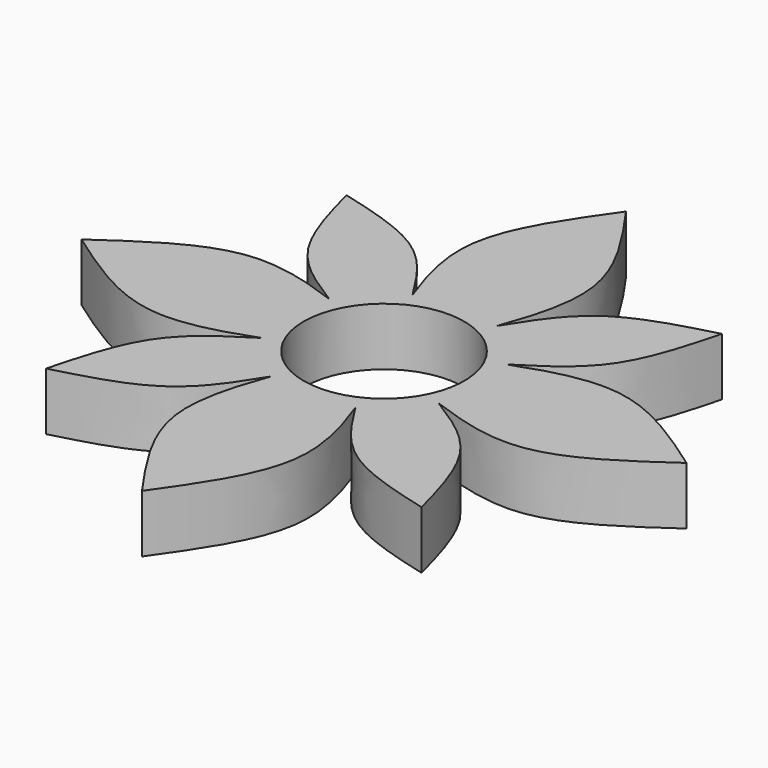
from build123d import *

# Parameters (mm, degrees)
F1_DEPTH = 8
F3_D     = 22.25


with BuildPart() as f1:
    # F0 (on Top) → F1 (new body)
    with BuildSketch(Plane.XY):
        with BuildLine():
            ThreePointArc((9.9471375726, 4.9819754226), (7.8665088435, 7.8666170375), (4.9818386126, 9.9472060921))
            ThreePointArc((4.9818386126, 9.9472060921), (0, 11.125), (-4.9818386126, 9.9472060921))
            ThreePointArc((-4.9818386126, 9.9472060921), (-7.8665088435, 7.8666170375), (-9.9471375726, 4.9819754226))
            ThreePointArc((-9.9471375726, 4.9819754226), (-11.125, 0), (-9.9471375726, -4.9819754226))
            ThreePointArc((-9.9471375726, -4.9819754226), (-7.8665088435, -7.8666170375), (-4.9818386126, -9.9472060921))
            ThreePointArc((-4.9818386126, -9.9472060921), (0, -11.125), (4.9818386126, -9.9472060921))
            ThreePointArc((4.9818386126, -9.9472060921), (7.8665088435, -7.8666170375), (9.9471375726, -4.9819754226))
            ThreePointArc((9.9471375726, -4.9819754226), (10.8265306192, -2.5596600853), (11.125, 0))
            ThreePointArc((11.125, 0), (10.8265306192, 2.5596600853), (9.9471375726, 4.9819754226))
        make_face()
        with BuildLine():
            add(Edge.make_bspline(
                [(4.9818386126, 9.9472060921), (5.2692870464, 10.7123686961), (5.5568645372, 11.4776931218), (5.8364125218, 12.242766493)],
                knots=[0, 0, 0, 0, 0.0701678859, 0.0701678859, 0.0701678859, 0.0701678859], degree=3))
            ThreePointArc((4.9818386126, 9.9472060921), (7.8665088435, 7.8666170375), (9.9471375726, 4.9819754226))
            add(Edge.make_bspline(
                [(9.9471375726, 4.9819754226), (10.7123016854, 5.2694244447), (11.4776275551, 5.5570012299), (12.2427023029, 5.8365471685)],
                knots=[1.11321e-05, 1.11321e-05, 1.11321e-05, 1.11321e-05, 0.0701791516, 0.0701791516, 0.0701791516, 0.0701791516], degree=3))
            ThreePointArc((12.2427023029, 5.8365471685), (9.5902820459, 9.5903875212), (5.8364125218, 12.242766493))
        make_face()
        with BuildLine():
            ThreePointArc((-4.9818386126, 9.9472060921), (0, 11.125), (4.9818386126, 9.9472060921))
            add(Edge.make_bspline(
                [(4.9818386126, 9.9472060921), (5.2692870464, 10.7123686961), (5.5568645372, 11.4776931218), (5.8364125218, 12.242766493)],
                knots=[0, 0, 0, 0, 0.0701678859, 0.0701678859, 0.0701678859, 0.0701678859], degree=3))
            ThreePointArc((5.8364125218, 12.242766493), (0, 13.5627815188), (-5.8364125218, 12.242766493))
            add(Edge.make_bspline(
                [(-4.9818386126, 9.9472060921), (-5.2692870464, 10.7123686961), (-5.5568645372, 11.4776931218), (-5.8364125218, 12.242766493)],
                knots=[0, 0, 0, 0, 0.0701678859, 0.0701678859, 0.0701678859, 0.0701678859], degree=3))
        make_face()
        with BuildLine():
            ThreePointArc((-9.9471375726, 4.9819754226), (-7.8665088435, 7.8666170375), (-4.9818386126, 9.9472060921))
            add(Edge.make_bspline(
                [(-4.9818386126, 9.9472060921), (-5.2692870464, 10.7123686961), (-5.5568645372, 11.4776931218), (-5.8364125218, 12.242766493)],
                knots=[0, 0, 0, 0, 0.0701678859, 0.0701678859, 0.0701678859, 0.0701678859], degree=3))
            ThreePointArc((-5.8364125218, 12.242766493), (-9.5902820459, 9.5903875212), (-12.2427023029, 5.8365471685))
            add(Edge.make_bspline(
                [(-9.9471375726, 4.9819754226), (-10.7123016854, 5.2694244447), (-11.4776275551, 5.5570012299), (-12.2427023029, 5.8365471685)],
                knots=[1.11321e-05, 1.11321e-05, 1.11321e-05, 1.11321e-05, 0.0701791516, 0.0701791516, 0.0701791516, 0.0701791516], degree=3))
        make_face()
        with BuildLine():
            add(Edge.make_bspline(
                [(9.9471375726, 4.9819754226), (10.7123016854, 5.2694244447), (11.4776275551, 5.5570012299), (12.2427023029, 5.8365471685)],
                knots=[1.11321e-05, 1.11321e-05, 1.11321e-05, 1.11321e-05, 0.0701791516, 0.0701791516, 0.0701791516, 0.0701791516], degree=3))
            ThreePointArc((9.9471375726, 4.9819754226), (10.8265306192, 2.5596600853), (11.125, 0))
            ThreePointArc((11.125, 0), (10.8265306192, -2.5596600853), (9.9471375726, -4.9819754226))
            add(Edge.make_bspline(
                [(9.9471375726, -4.9819754226), (10.7123016854, -5.2694244447), (11.4776275551, -5.5570012299), (12.2427023029, -5.8365471685)],
                knots=[1.11321e-05, 1.11321e-05, 1.11321e-05, 1.11321e-05, 0.0701791516, 0.0701791516, 0.0701791516, 0.0701791516], degree=3))
            ThreePointArc((12.2427023029, -5.8365471685), (12.2428068623, -5.8363278403), (12.2429114178, -5.8361085102))
            ThreePointArc((12.2429114178, -5.8361085102), (13.2286993926, -2.9917478013), (13.5627815188, 0))
            ThreePointArc((13.5627815188, 0), (13.2286993926, 2.9917478013), (12.2429114178, 5.8361085102))
            ThreePointArc((12.2429114178, 5.8361085102), (12.2428068623, 5.8363278403), (12.2427023029, 5.8365471685))
        make_face()
        with BuildLine():
            ThreePointArc((-5.8364125218, 12.242766493), (0, 13.5627815188), (5.8364125218, 12.242766493))
            add(Edge.make_bspline(
                [(5.8364125218, 12.242766493), (7.4881688325, 16.7633312564), (10.5639067692, 26.8820696151), (3.7644701713, 36.5283294837), (0, 41.8734326959)],
                knots=[0.0701678859, 0.0701678859, 0.0701678859, 0.0701678859, 0.484766648, 1, 1, 1, 1], degree=3))
            add(Edge.make_bspline(
                [(-5.8364125218, 12.242766493), (-7.4881688325, 16.7633312564), (-10.5639067692, 26.8820696151), (-3.7644701713, 36.5283294837), (0, 41.8734326959)],
                knots=[0.0701678859, 0.0701678859, 0.0701678859, 0.0701678859, 0.484766648, 1, 1, 1, 1], degree=3))
        make_face()
        Polygon((2.4637663324, 30.8732958237), (5.4101836661, 26.3272686725), (2.9464173337, 21.5025828357), (-2.4637663324, 21.2239241501), (-5.4101836661, 25.7699513014), (-2.9464173337, 30.5946371381), align=None, mode=Mode.SUBTRACT)
        with BuildLine():
            add(Edge.make_bspline(
                [(5.8364125218, 12.242766493), (7.8640126159, 15.4827332927), (12.1444054008, 22.3225093182), (21.2142960732, 24.7235177216), (25.987826083, 25.9871807669)],
                knots=[0, 0, 0, 0, 0.4736948677, 1, 1, 1, 1], degree=3))
            ThreePointArc((5.8364125218, 12.242766493), (9.5902820459, 9.5903875212), (12.2427023029, 5.8365471685))
            add(Edge.make_bspline(
                [(12.2427023029, 5.8365471685), (12.2434313303, 5.8368135433), (12.2441603575, 5.8370799108), (12.2448893845, 5.8373462711)],
                knots=[0.0701791516, 0.0701791516, 0.0701791516, 0.0701791516, 0.0702460136, 0.0702460136, 0.0702460136, 0.0702460136], degree=3))
            add(Edge.make_bspline(
                [(12.2448893845, 5.8373462711), (15.4842471687, 7.8644533679), (22.3230423426, 12.1447253647), (24.7240445028, 21.2136821375), (25.987826083, 25.9871807669)],
                knots=[9.63938e-05, 9.63938e-05, 9.63938e-05, 9.63938e-05, 0.4736948677, 1, 1, 1, 1], degree=3))
        make_face()
        with BuildLine():
            ThreePointArc((-9.9471375726, -4.9819754226), (-11.125, 0), (-9.9471375726, 4.9819754226))
            add(Edge.make_bspline(
                [(-9.9471375726, 4.9819754226), (-10.7123016854, 5.2694244447), (-11.4776275551, 5.5570012299), (-12.2427023029, 5.8365471685)],
                knots=[1.11321e-05, 1.11321e-05, 1.11321e-05, 1.11321e-05, 0.0701791516, 0.0701791516, 0.0701791516, 0.0701791516], degree=3))
            ThreePointArc((-12.2427023029, 5.8365471685), (-12.2428068623, 5.8363278403), (-12.2429114178, 5.8361085102))
            ThreePointArc((-12.2429114178, 5.8361085102), (-13.5627815188, 0), (-12.2429114178, -5.8361085102))
            ThreePointArc((-12.2429114178, -5.8361085102), (-12.2428068623, -5.8363278403), (-12.2427023029, -5.8365471685))
            add(Edge.make_bspline(
                [(-9.9471375726, -4.9819754226), (-10.7123016854, -5.2694244447), (-11.4776275551, -5.5570012299), (-12.2427023029, -5.8365471685)],
                knots=[1.11321e-05, 1.11321e-05, 1.11321e-05, 1.11321e-05, 0.0701791516, 0.0701791516, 0.0701791516, 0.0701791516], degree=3))
        make_face()
        with BuildLine():
            ThreePointArc((-12.2427023029, 5.8365471685), (-9.5902820459, 9.5903875212), (-5.8364125218, 12.242766493))
            add(Edge.make_bspline(
                [(-5.8364125218, 12.242766493), (-7.8640126159, 15.4827332927), (-12.1444054008, 22.3225093182), (-21.2142960732, 24.7235177216), (-25.987826083, 25.9871807669)],
                knots=[0, 0, 0, 0, 0.4736948677, 1, 1, 1, 1], degree=3))
            add(Edge.make_bspline(
                [(-12.2448893845, 5.8373462711), (-15.4842471687, 7.8644533679), (-22.3230423426, 12.1447253647), (-24.7240445028, 21.2136821375), (-25.987826083, 25.9871807669)],
                knots=[9.63938e-05, 9.63938e-05, 9.63938e-05, 9.63938e-05, 0.4736948677, 1, 1, 1, 1], degree=3))
            add(Edge.make_bspline(
                [(-12.2427023029, 5.8365471685), (-12.2434313303, 5.8368135433), (-12.2441603575, 5.8370799108), (-12.2448893845, 5.8373462711)],
                knots=[0.0701791516, 0.0701791516, 0.0701791516, 0.0701791516, 0.0702460136, 0.0702460136, 0.0702460136, 0.0702460136], degree=3))
        make_face()
        with BuildLine():
            add(Edge.make_bspline(
                [(12.2427023029, 5.8365471685), (12.2434313303, 5.8368135433), (12.2441603575, 5.8370799108), (12.2448893845, 5.8373462711)],
                knots=[0.0701791516, 0.0701791516, 0.0701791516, 0.0701791516, 0.0702460136, 0.0702460136, 0.0702460136, 0.0702460136], degree=3))
            ThreePointArc((12.2427023029, 5.8365471685), (12.2428068623, 5.8363278403), (12.2429114178, 5.8361085102))
            add(Edge.make_bspline(
                [(12.2429114178, 5.8361085102), (12.24357074, 5.8365210972), (12.2442300623, 5.8369336841), (12.2448893845, 5.8373462711)],
                knots=[0, 0, 0, 0, 9.63938e-05, 9.63938e-05, 9.63938e-05, 9.63938e-05], degree=3))
        make_face()
        with BuildLine():
            ThreePointArc((-4.9818386126, -9.9472060921), (-7.8665088435, -7.8666170375), (-9.9471375726, -4.9819754226))
            add(Edge.make_bspline(
                [(-9.9471375726, -4.9819754226), (-10.7123016854, -5.2694244447), (-11.4776275551, -5.5570012299), (-12.2427023029, -5.8365471685)],
                knots=[1.11321e-05, 1.11321e-05, 1.11321e-05, 1.11321e-05, 0.0701791516, 0.0701791516, 0.0701791516, 0.0701791516], degree=3))
            ThreePointArc((-12.2427023029, -5.8365471685), (-9.5902820459, -9.5903875212), (-5.8364125218, -12.242766493))
            add(Edge.make_bspline(
                [(-4.9818386126, -9.9472060921), (-5.2692870464, -10.7123686961), (-5.5568645372, -11.4776931218), (-5.8364125218, -12.242766493)],
                knots=[0, 0, 0, 0, 0.0701678859, 0.0701678859, 0.0701678859, 0.0701678859], degree=3))
        make_face()
        with BuildLine():
            ThreePointArc((-12.2429114178, 5.8361085102), (-12.2428068623, 5.8363278403), (-12.2427023029, 5.8365471685))
            add(Edge.make_bspline(
                [(-12.2427023029, 5.8365471685), (-12.2434313303, 5.8368135433), (-12.2441603575, 5.8370799108), (-12.2448893845, 5.8373462711)],
                knots=[0.0701791516, 0.0701791516, 0.0701791516, 0.0701791516, 0.0702460136, 0.0702460136, 0.0702460136, 0.0702460136], degree=3))
            add(Edge.make_bspline(
                [(-12.2429114178, 5.8361085102), (-12.24357074, 5.8365210972), (-12.2442300623, 5.8369336841), (-12.2448893845, 5.8373462711)],
                knots=[0, 0, 0, 0, 9.63938e-05, 9.63938e-05, 9.63938e-05, 9.63938e-05], degree=3))
        make_face()
        with BuildLine():
            add(Edge.make_bspline(
                [(9.9471375726, -4.9819754226), (10.7123016854, -5.2694244447), (11.4776275551, -5.5570012299), (12.2427023029, -5.8365471685)],
                knots=[1.11321e-05, 1.11321e-05, 1.11321e-05, 1.11321e-05, 0.0701791516, 0.0701791516, 0.0701791516, 0.0701791516], degree=3))
            ThreePointArc((9.9471375726, -4.9819754226), (7.8665088435, -7.8666170375), (4.9818386126, -9.9472060921))
            add(Edge.make_bspline(
                [(4.9818386126, -9.9472060921), (5.2692870464, -10.7123686961), (5.5568645372, -11.4776931218), (5.8364125218, -12.242766493)],
                knots=[0, 0, 0, 0, 0.0701678859, 0.0701678859, 0.0701678859, 0.0701678859], degree=3))
            ThreePointArc((5.8364125218, -12.242766493), (9.5902820459, -9.5903875212), (12.2427023029, -5.8365471685))
        make_face()
        with BuildLine():
            add(Edge.make_bspline(
                [(12.2448893845, 5.8373462711), (16.7645989794, 7.4886856309), (26.8824474311, 10.5633354573), (36.5278967878, 3.7644701713), (41.873, 0)],
                knots=[0.0702460136, 0.0702460136, 0.0702460136, 0.0702460136, 0.484766648, 1, 1, 1, 1], degree=3))
            add(Edge.make_bspline(
                [(12.2429114178, 5.8361085102), (12.24357074, 5.8365210972), (12.2442300623, 5.8369336841), (12.2448893845, 5.8373462711)],
                knots=[0, 0, 0, 0, 9.63938e-05, 9.63938e-05, 9.63938e-05, 9.63938e-05], degree=3))
            ThreePointArc((12.2429114178, 5.8361085102), (13.2286993926, 2.9917478013), (13.5627815188, 0))
            ThreePointArc((13.5627815188, 0), (13.2286993926, -2.9917478013), (12.2429114178, -5.8361085102))
            add(Edge.make_bspline(
                [(12.2429114178, -5.8361085102), (12.24357074, -5.8365210972), (12.2442300623, -5.8369336841), (12.2448893845, -5.8373462711)],
                knots=[0, 0, 0, 0, 9.63938e-05, 9.63938e-05, 9.63938e-05, 9.63938e-05], degree=3))
            add(Edge.make_bspline(
                [(12.2448893845, -5.8373462711), (16.7645989794, -7.4886856309), (26.8824474311, -10.5633354573), (36.5278967878, -3.7644701713), (41.873, 0)],
                knots=[0.0702460136, 0.0702460136, 0.0702460136, 0.0702460136, 0.484766648, 1, 1, 1, 1], degree=3))
        make_face()
        Polygon((25.7699513014, 5.4101836661), (30.5946371381, 2.9464173337), (30.8732958237, -2.4637663324), (26.3272686725, -5.4101836661), (21.5025828357, -2.9464173337), (21.2239241501, 2.4637663324), align=None, mode=Mode.SUBTRACT)
        with BuildLine():
            ThreePointArc((4.9818386126, -9.9472060921), (0, -11.125), (-4.9818386126, -9.9472060921))
            add(Edge.make_bspline(
                [(-4.9818386126, -9.9472060921), (-5.2692870464, -10.7123686961), (-5.5568645372, -11.4776931218), (-5.8364125218, -12.242766493)],
                knots=[0, 0, 0, 0, 0.0701678859, 0.0701678859, 0.0701678859, 0.0701678859], degree=3))
            ThreePointArc((-5.8364125218, -12.242766493), (0, -13.5627815188), (5.8364125218, -12.242766493))
            add(Edge.make_bspline(
                [(4.9818386126, -9.9472060921), (5.2692870464, -10.7123686961), (5.5568645372, -11.4776931218), (5.8364125218, -12.242766493)],
                knots=[0, 0, 0, 0, 0.0701678859, 0.0701678859, 0.0701678859, 0.0701678859], degree=3))
        make_face()
        with BuildLine():
            ThreePointArc((-5.8364125218, -12.242766493), (-9.5902820459, -9.5903875212), (-12.2427023029, -5.8365471685))
            add(Edge.make_bspline(
                [(-12.2427023029, -5.8365471685), (-12.2434313303, -5.8368135433), (-12.2441603575, -5.8370799108), (-12.2448893845, -5.8373462711)],
                knots=[0.0701791516, 0.0701791516, 0.0701791516, 0.0701791516, 0.0702460136, 0.0702460136, 0.0702460136, 0.0702460136], degree=3))
            add(Edge.make_bspline(
                [(-12.2448893845, -5.8373462711), (-15.4842471687, -7.8644533679), (-22.3230423426, -12.1447253647), (-24.7240445028, -21.2136821375), (-25.987826083, -25.9871807669)],
                knots=[9.63938e-05, 9.63938e-05, 9.63938e-05, 9.63938e-05, 0.4736948677, 1, 1, 1, 1], degree=3))
            add(Edge.make_bspline(
                [(-5.8364125218, -12.242766493), (-7.8640126159, -15.4827332927), (-12.1444054008, -22.3225093182), (-21.2142960732, -24.7235177216), (-25.987826083, -25.9871807669)],
                knots=[0, 0, 0, 0, 0.4736948677, 1, 1, 1, 1], degree=3))
        make_face()
        with BuildLine():
            add(Edge.make_bspline(
                [(-12.2427023029, -5.8365471685), (-12.2434313303, -5.8368135433), (-12.2441603575, -5.8370799108), (-12.2448893845, -5.8373462711)],
                knots=[0.0701791516, 0.0701791516, 0.0701791516, 0.0701791516, 0.0702460136, 0.0702460136, 0.0702460136, 0.0702460136], degree=3))
            ThreePointArc((-12.2427023029, -5.8365471685), (-12.2428068623, -5.8363278403), (-12.2429114178, -5.8361085102))
            add(Edge.make_bspline(
                [(-12.2429114178, -5.8361085102), (-12.24357074, -5.8365210972), (-12.2442300623, -5.8369336841), (-12.2448893845, -5.8373462711)],
                knots=[0, 0, 0, 0, 9.63938e-05, 9.63938e-05, 9.63938e-05, 9.63938e-05], degree=3))
        make_face()
        with BuildLine():
            add(Edge.make_bspline(
                [(-12.2429114178, 5.8361085102), (-12.24357074, 5.8365210972), (-12.2442300623, 5.8369336841), (-12.2448893845, 5.8373462711)],
                knots=[0, 0, 0, 0, 9.63938e-05, 9.63938e-05, 9.63938e-05, 9.63938e-05], degree=3))
            add(Edge.make_bspline(
                [(-12.2448893845, 5.8373462711), (-16.7645989794, 7.4886856309), (-26.8824474311, 10.5633354573), (-36.5278967878, 3.7644701713), (-41.873, 0)],
                knots=[0.0702460136, 0.0702460136, 0.0702460136, 0.0702460136, 0.484766648, 1, 1, 1, 1], degree=3))
            add(Edge.make_bspline(
                [(-12.2448893845, -5.8373462711), (-16.7645989794, -7.4886856309), (-26.8824474311, -10.5633354573), (-36.5278967878, -3.7644701713), (-41.873, 0)],
                knots=[0.0702460136, 0.0702460136, 0.0702460136, 0.0702460136, 0.484766648, 1, 1, 1, 1], degree=3))
            add(Edge.make_bspline(
                [(-12.2429114178, -5.8361085102), (-12.24357074, -5.8365210972), (-12.2442300623, -5.8369336841), (-12.2448893845, -5.8373462711)],
                knots=[0, 0, 0, 0, 9.63938e-05, 9.63938e-05, 9.63938e-05, 9.63938e-05], degree=3))
            ThreePointArc((-12.2429114178, -5.8361085102), (-13.5627815188, 0), (-12.2429114178, 5.8361085102))
        make_face()
        Polygon((-25.7699513014, -5.4101836661), (-30.5946371381, -2.9464173337), (-30.8732958237, 2.4637663324), (-26.3272686725, 5.4101836661), (-21.5025828357, 2.9464173337), (-21.2239241501, -2.4637663324), align=None, mode=Mode.SUBTRACT)
        with BuildLine():
            ThreePointArc((12.2429114178, -5.8361085102), (12.2428068623, -5.8363278403), (12.2427023029, -5.8365471685))
            add(Edge.make_bspline(
                [(12.2427023029, -5.8365471685), (12.2434313303, -5.8368135433), (12.2441603575, -5.8370799108), (12.2448893845, -5.8373462711)],
                knots=[0.0701791516, 0.0701791516, 0.0701791516, 0.0701791516, 0.0702460136, 0.0702460136, 0.0702460136, 0.0702460136], degree=3))
            add(Edge.make_bspline(
                [(12.2429114178, -5.8361085102), (12.24357074, -5.8365210972), (12.2442300623, -5.8369336841), (12.2448893845, -5.8373462711)],
                knots=[0, 0, 0, 0, 9.63938e-05, 9.63938e-05, 9.63938e-05, 9.63938e-05], degree=3))
        make_face()
        with BuildLine():
            add(Edge.make_bspline(
                [(12.2427023029, -5.8365471685), (12.2434313303, -5.8368135433), (12.2441603575, -5.8370799108), (12.2448893845, -5.8373462711)],
                knots=[0.0701791516, 0.0701791516, 0.0701791516, 0.0701791516, 0.0702460136, 0.0702460136, 0.0702460136, 0.0702460136], degree=3))
            ThreePointArc((12.2427023029, -5.8365471685), (9.5902820459, -9.5903875212), (5.8364125218, -12.242766493))
            add(Edge.make_bspline(
                [(5.8364125218, -12.242766493), (7.8640126159, -15.4827332927), (12.1444054008, -22.3225093182), (21.2142960732, -24.7235177216), (25.987826083, -25.9871807669)],
                knots=[0, 0, 0, 0, 0.4736948677, 1, 1, 1, 1], degree=3))
            add(Edge.make_bspline(
                [(12.2448893845, -5.8373462711), (15.4842471687, -7.8644533679), (22.3230423426, -12.1447253647), (24.7240445028, -21.2136821375), (25.987826083, -25.9871807669)],
                knots=[9.63938e-05, 9.63938e-05, 9.63938e-05, 9.63938e-05, 0.4736948677, 1, 1, 1, 1], degree=3))
        make_face()
        with BuildLine():
            ThreePointArc((5.8364125218, -12.242766493), (0, -13.5627815188), (-5.8364125218, -12.242766493))
            add(Edge.make_bspline(
                [(-5.8364125218, -12.242766493), (-7.4881688325, -16.7633312564), (-10.5639067692, -26.8820696151), (-3.7644701713, -36.5283294837), (0, -41.8734326959)],
                knots=[0.0701678859, 0.0701678859, 0.0701678859, 0.0701678859, 0.484766648, 1, 1, 1, 1], degree=3))
            add(Edge.make_bspline(
                [(5.8364125218, -12.242766493), (7.4881688325, -16.7633312564), (10.5639067692, -26.8820696151), (3.7644701713, -36.5283294837), (0, -41.8734326959)],
                knots=[0.0701678859, 0.0701678859, 0.0701678859, 0.0701678859, 0.484766648, 1, 1, 1, 1], degree=3))
        make_face()
        Polygon((5.4101836661, -25.7699513014), (2.9464173337, -30.5946371381), (-2.4637663324, -30.8732958237), (-5.4101836661, -26.3272686725), (-2.9464173337, -21.5025828357), (2.4637663324, -21.2239241501), align=None, mode=Mode.SUBTRACT)
        Polygon((2.9464173337, 21.5025828357), (5.4101836661, 26.3272686725), (2.4637663324, 30.8732958237), (-2.9464173337, 30.5946371381), (-5.4101836661, 25.7699513014), (-2.4637663324, 21.2239241501), align=None)
        Polygon((-30.8732958237, 2.4637663324), (-30.5946371381, -2.9464173337), (-25.7699513014, -5.4101836661), (-21.2239241501, -2.4637663324), (-21.5025828357, 2.9464173337), (-26.3272686725, 5.4101836661), align=None)
        Polygon((-2.4637663324, -30.8732958237), (2.9464173337, -30.5946371381), (5.4101836661, -25.7699513014), (2.4637663324, -21.2239241501), (-2.9464173337, -21.5025828357), (-5.4101836661, -26.3272686725), align=None)
        Polygon((30.8732958237, -2.4637663324), (30.5946371381, 2.9464173337), (25.7699513014, 5.4101836661), (21.2239241501, 2.4637663324), (21.5025828357, -2.9464173337), (26.3272686725, -5.4101836661), align=None)
    extrude(amount=F1_DEPTH)

    # F3 (through all)
    with Locations(Plane(origin=(0, 0, 0), x_dir=(1, 0, 0), z_dir=(0, 0, -1))):
        with Locations((0, 0)):
            Hole(F3_D / 2)


solid = f1.part
